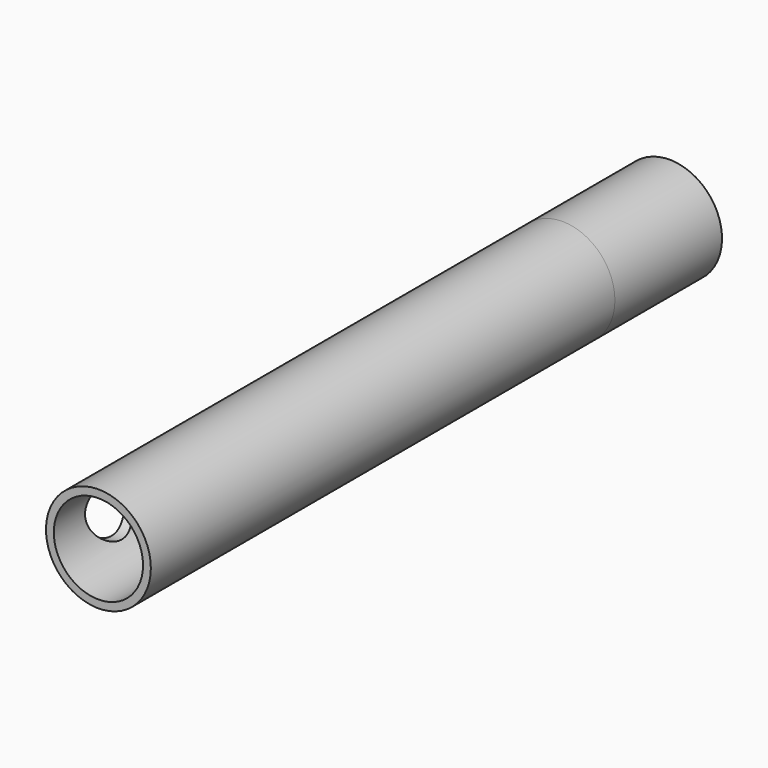
from build123d import *

# Parameters (mm, degrees)
F3_R      = 4.7
F4_DEPTH  = 42
F8_DEPTH  = 42
F6_R      = 4.7
F6_R_2    = 4
F9_DEPTH  = 10
F7_R      = 4.7
F7_R_2    = 4
F10_DEPTH = 12
F11_R     = 2.75
F12_DEPTH = 4.701


# Not quite as in the source:
# - ends of sketch curves that miss each other by under 0.0002 mm in the source are joined


with BuildPart() as f4:
    # F3 (on Front) → F4 (new body)
    with BuildSketch(Plane.XZ):
        Circle(F3_R)
    extrude(amount=F4_DEPTH)

    # F5 (on face) → F8 (cut, through all)
    with BuildSketch(Plane.XZ.offset(42)):
        with BuildLine():
            Line((-1.25, -3.8), (0, -3.8))
            Line((0, -3.8), (1.25, -3.8))
            Line((1.25, -3.8), (1.25, -3.7))
            ThreePointArc((1.25, -3.7), (1.3085786438, -3.5585786438), (1.45, -3.5))
            Line((1.45, -3.5), (2, -3.5))
            Line((2, -3.5), (2, -3.05))
            ThreePointArc((2, -3.05), (2.0585786438, -2.9085786438), (2.2, -2.85))
            Line((2.2, -2.85), (3.15, -2.85))
            Line((3.15, -2.85), (3.15, -2.15))
            Line((3.15, -2.15), (2.2, -2.15))
            ThreePointArc((2.2, -2.15), (2.0585786438, -2.0914213562), (2, -1.95))
            Line((2, -1.95), (2, -1.887459))
            ThreePointArc((2, -1.887459), (2.1033535752, -1.771554046), (2.2, -1.65))
            Line((2.2, -1.65), (3.75, -1.65))
            Line((3.75, -1.65), (3.75, 0))
            Line((3.75, 0), (3.75, 1.65))
            Line((3.75, 1.65), (2.2, 1.65))
            ThreePointArc((2.2, 1.65), (2.1033535752, 1.771554046), (1.9999998047, 1.8874588157))
            Line((1.9999998047, 1.8874588157), (2, 1.95))
            ThreePointArc((2, 1.95), (2.0585786438, 2.0914213562), (2.2, 2.15))
            Line((2.2, 2.15), (3.15, 2.15))
            Line((3.15, 2.15), (3.15, 2.85))
            Line((3.15, 2.85), (2.2, 2.85))
            ThreePointArc((2.2, 2.85), (2.0585786438, 2.9085786438), (2, 3.05))
            Line((2, 3.05), (2, 3.5))
            Line((2, 3.5), (1.45, 3.5))
            ThreePointArc((1.45, 3.5), (1.3085786438, 3.5585786438), (1.25, 3.7))
            Line((1.25, 3.7), (1.25, 3.8))
            Line((1.25, 3.8), (0, 3.8))
            Line((0, 3.8), (-1.25, 3.8))
            Line((-1.25, 3.8), (-1.25, 3.7))
            ThreePointArc((-1.25, 3.7), (-1.3085786438, 3.5585786438), (-1.45, 3.5))
            Line((-1.45, 3.5), (-2, 3.5))
            Line((-2, 3.5), (-2, 3.05))
            ThreePointArc((-2, 3.05), (-2.0585786438, 2.9085786438), (-2.2, 2.85))
            Line((-2.2, 2.85), (-3.15, 2.85))
            Line((-3.15, 2.85), (-3.15, 2.15))
            Line((-3.15, 2.15), (-2.2, 2.15))
            ThreePointArc((-2.2, 2.15), (-2.0585786438, 2.0914213562), (-2, 1.95))
            Line((-2, 1.95), (-2, 1.887459))
            ThreePointArc((-2, 1.887459), (-2.1033535752, 1.771554046), (-2.2, 1.65))
            Line((-2.2, 1.65), (-3.75, 1.65))
            Line((-3.75, 1.65), (-3.75, 0))
            Line((-3.75, 0), (-3.75, -1.65))
            Line((-3.75, -1.65), (-2.2, -1.65))
            ThreePointArc((-2.2, -1.65), (-2.1033535752, -1.771554046), (-1.9999998047, -1.8874588157))
            Line((-1.9999998047, -1.8874588157), (-2, -1.95))
            ThreePointArc((-2, -1.95), (-2.0585786438, -2.0914213562), (-2.2, -2.15))
            Line((-2.2, -2.15), (-3.15, -2.15))
            Line((-3.15, -2.15), (-3.15, -2.85))
            Line((-3.15, -2.85), (-2.2, -2.85))
            ThreePointArc((-2.2, -2.85), (-2.0585786438, -2.9085786438), (-2, -3.05))
            Line((-2, -3.05), (-2, -3.5))
            Line((-2, -3.5), (-1.45, -3.5))
            ThreePointArc((-1.45, -3.5), (-1.3085786438, -3.5585786438), (-1.25, -3.7))
            Line((-1.25, -3.7), (-1.25, -3.8))
        make_face()
    extrude(amount=-F8_DEPTH, mode=Mode.SUBTRACT)

    # F6 (on face) → F9 (join)
    with BuildSketch(Plane.XZ.offset(42)):
        Circle(F6_R)
        Circle(F6_R_2, mode=Mode.SUBTRACT)
    extrude(amount=F9_DEPTH)

    # F7 (on face) → F10 (join)
    with BuildSketch(Plane(origin=(0, 0, 0), x_dir=(-1, 0, 0), z_dir=(0, 1, 0))):
        Circle(F7_R)
        Circle(F7_R_2, mode=Mode.SUBTRACT)
    extrude(amount=F10_DEPTH)

    # F11 (on Right) → F12 (cut, through all)
    with BuildSketch(Plane.YZ):
        with Locations((-45.75, 0)):
            Circle(F11_R)
    extrude(amount=-F12_DEPTH, mode=Mode.SUBTRACT)


solid = f4.part
